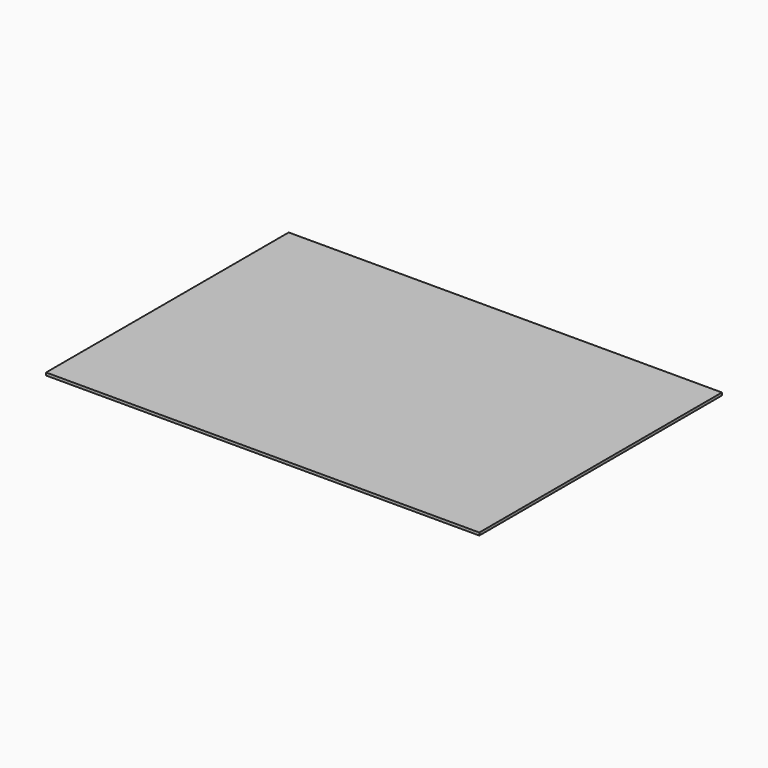
from build123d import *

# Parameters (mm, degrees)
F0_W     = 762
F0_H     = 533.4
F1_DEPTH = 4.7625


# Not quite as in the source:
# - a length typed as a fraction of an inch, garbled in the dataset ("3 / 203.2 mm" for 3/8 in), is restored


with BuildPart() as f1:
    # F0 (on Top) → F1 (new body)
    with BuildSketch(Plane.XY):
        with Locations((231.4390618205, 225.2508450184)):
            Rectangle(F0_W, F0_H)
    extrude(amount=-F1_DEPTH)


solid = f1.part
